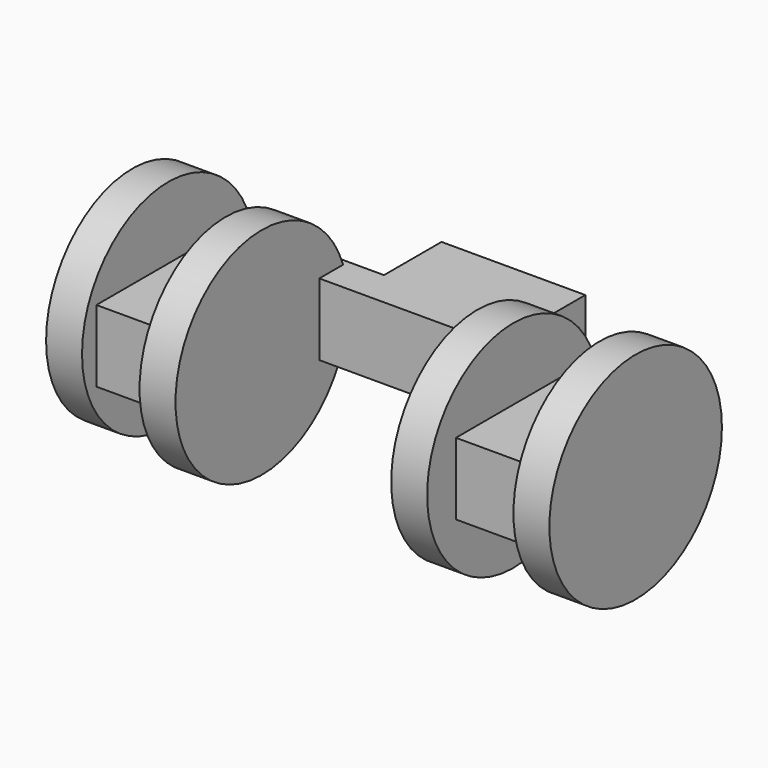
from build123d import *

# Parameters (mm, degrees)
F0_W      = 12.7
F0_H      = 6.35
F1_DEPTH  = 6.35
F2_W      = 12.7
F2_H      = 6.35
F3_DEPTH  = 3.175
F4_W      = 6.35
F4_H      = 6.35
F5_DEPTH  = 12.7
F6_R      = 9.525
F6_W      = 15.875
F6_H      = 6.35
F7_DEPTH  = 3.175
F8_R      = 9.525
F9_DEPTH  = 3.175
F10_R     = 9.525
F11_DEPTH = 3.175
F12_R     = 9.525
F13_DEPTH = 3.175


# Not quite as in the source:
# - a feature names something its author has since deleted; it is built from what else it names


with BuildPart() as f1:
    # F0 (on Front) → F1 (new body)
    with BuildSketch(Plane.XZ):
        with Locations((6.35, 3.175)):
            Rectangle(F0_W, F0_H)
    extrude(amount=F1_DEPTH)

    # F2 (on face) → F3 (join)
    with BuildSketch(Plane.XZ.offset(6.35)):
        with Locations((-6.35, 3.175)):
            Rectangle(F2_W, F2_H)
        with Locations((6.35, 3.175)):
            Rectangle(F2_W, F2_H)
        with Locations((19.05, 3.175)):
            Rectangle(F2_W, F2_H)
    extrude(amount=F3_DEPTH)

    # F4 (on face) → F5 (join)
    with BuildSketch(Plane.XZ.offset(9.525)):
        with Locations((-9.525, 3.175)):
            Rectangle(F4_W, F4_H)
        with Locations((22.225, 3.175)):
            Rectangle(F4_W, F4_H)
    extrude(amount=F5_DEPTH)

    # F6 (on face) → F7 (join)
    with BuildSketch(Plane.YZ.offset(25.4)):
        with Locations((-14.2875, 3.175)):
            Circle(F6_R)
        with Locations((-14.2875, 3.175)):
            Rectangle(F6_W, F6_H, mode=Mode.SUBTRACT)
        with Locations((-14.2875, 3.175)):
            Rectangle(F6_W, F6_H)
    extrude(amount=F7_DEPTH)

    # F8 (on face) → F9 (join)
    with BuildSketch(Plane(origin=(-12.7, 0, 0), x_dir=(0, -1, 0), z_dir=(-1, 0, 0))):
        with Locations((14.2875, 3.175)):
            Circle(F8_R)
    extrude(amount=F9_DEPTH)

    # F10 (on face) → F11 (join)
    with BuildSketch(Plane(origin=(19.05, 0, 0), x_dir=(0, -1, 0), z_dir=(-1, 0, 0))):
        with Locations((15.875, 3.175)):
            Circle(F10_R)
    extrude(amount=F11_DEPTH)

    # F12 (on face) → F13 (join)
    with BuildSketch(Plane.YZ.offset(-6.35)):
        with Locations((-15.875, 3.175)):
            Circle(F12_R)
    extrude(amount=F13_DEPTH)


solid = f1.part
